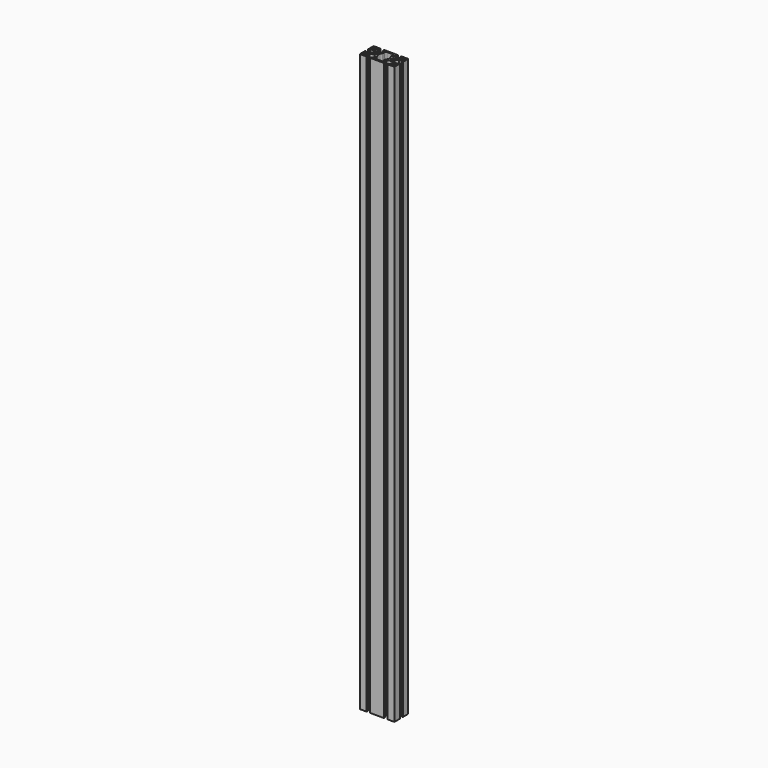
from build123d import *

# Parameters (mm, degrees)
F0_R     = 3
F0_R_2   = 2.5
F1_DEPTH = 1000
F2_R     = 2
F3_R     = 7


# Not quite as in the source:
# - a feature names something its author has since deleted; it is built from what else it names


with BuildPart() as f1:
    # F0 (on Top) → F1 (new body)
    with BuildSketch(Plane.XY):
        with BuildLine():
            Line((18.15, -15), (30, -15))
            Line((30, -15), (30, -3.15))
            Line((30, -3.15), (27.5, -3.15))
            Line((27.5, -3.15), (27.5, -5.15))
            Line((27.5, -5.15), (21.5477069044, -5.15))
            ThreePointArc((21.5477069044, -5.15), (19.5, 0), (21.5477069044, 5.15))
            Line((21.5477069044, 5.15), (27.5, 5.15))
            Line((27.5, 5.15), (27.5, 3.15))
            Line((27.5, 3.15), (30, 3.15))
            Line((30, 3.15), (30, 15))
            Line((30, 15), (18.15, 15))
            Line((18.15, 15), (18.15, 12.5))
            Line((18.15, 12.5), (20.15, 12.5))
            Line((20.15, 12.5), (20.15, 6.5477069044))
            ThreePointArc((20.15, 6.5477069044), (15, 4.5), (9.85, 6.5477069044))
            Line((9.85, 6.5477069044), (9.85, 12.5))
            Line((9.85, 12.5), (11.85, 12.5))
            Line((11.85, 12.5), (11.85, 15))
            Line((11.85, 15), (-11.85, 15))
            Line((-11.85, 15), (-11.85, 12.5))
            Line((-11.85, 12.5), (-9.85, 12.5))
            Line((-9.85, 12.5), (-9.85, 6.5477069044))
            ThreePointArc((-9.85, 6.5477069044), (-15, 4.5), (-20.15, 6.5477069044))
            Line((-20.15, 6.5477069044), (-20.15, 12.5))
            Line((-20.15, 12.5), (-18.15, 12.5))
            Line((-18.15, 12.5), (-18.15, 15))
            Line((-18.15, 15), (-30, 15))
            Line((-30, 15), (-30, 3.15))
            Line((-30, 3.15), (-27.5, 3.15))
            Line((-27.5, 3.15), (-27.5, 5.15))
            Line((-27.5, 5.15), (-21.5477069044, 5.15))
            ThreePointArc((-21.5477069044, 5.15), (-19.5, 0), (-21.5477069044, -5.15))
            Line((-21.5477069044, -5.15), (-27.5, -5.15))
            Line((-27.5, -5.15), (-27.5, -3.15))
            Line((-27.5, -3.15), (-30, -3.15))
            Line((-30, -3.15), (-30, -15))
            Line((-30, -15), (-18.15, -15))
            Line((-18.15, -15), (-18.15, -12.5))
            Line((-18.15, -12.5), (-20.15, -12.5))
            Line((-20.15, -12.5), (-20.15, -6.5477069044))
            ThreePointArc((-20.15, -6.5477069044), (-15, -4.5), (-9.85, -6.5477069044))
            Line((-9.85, -6.5477069044), (-9.85, -12.5))
            Line((-9.85, -12.5), (-11.85, -12.5))
            Line((-11.85, -12.5), (-11.85, -15))
            Line((-11.85, -15), (11.85, -15))
            Line((11.85, -15), (11.85, -12.5))
            Line((11.85, -12.5), (9.85, -12.5))
            Line((9.85, -12.5), (9.85, -6.5477069044))
            ThreePointArc((9.85, -6.5477069044), (15, -4.5), (20.15, -6.5477069044))
            Line((20.15, -6.5477069044), (20.15, -12.5))
            Line((20.15, -12.5), (18.15, -12.5))
            Line((18.15, -12.5), (18.15, -15))
        make_face()
        with Locations((-25, -10)):
            Circle(F0_R, mode=Mode.SUBTRACT)
        with Locations((25, -10)):
            Circle(F0_R, mode=Mode.SUBTRACT)
        with Locations((-15, 0)):
            Circle(F0_R_2, mode=Mode.SUBTRACT)
        with Locations((-25, 10)):
            Circle(F0_R, mode=Mode.SUBTRACT)
        Polygon((-7, 7), (-7, 12.5), (0, 12.5), (7, 12.5), (7, 7), (10, 0), (7, -7), (7, -12.5), (0, -12.5), (-7, -12.5), (-7, -7), (-10, 0), align=None, mode=Mode.SUBTRACT)
        with Locations((15, 0)):
            Circle(F0_R_2, mode=Mode.SUBTRACT)
        with Locations((25, 10)):
            Circle(F0_R, mode=Mode.SUBTRACT)
    extrude(amount=F1_DEPTH)

    # F2
    f2_edges = [f1.edges().sort_by_distance(p)[0] for p in [
        (-7, 12.5, 500),
        (7, 12.5, 500),
    ]]
    fillet(f2_edges, radius=F2_R)

    # F3
    f3_edges = [f1.edges().sort_by_distance(p)[0] for p in [
        (-7, 7, 500),
        (-10, 0, 500),
        (7, 7, 500),
        (10, 0, 500),
    ]]
    fillet(f3_edges, radius=F3_R)


solid = f1.part
